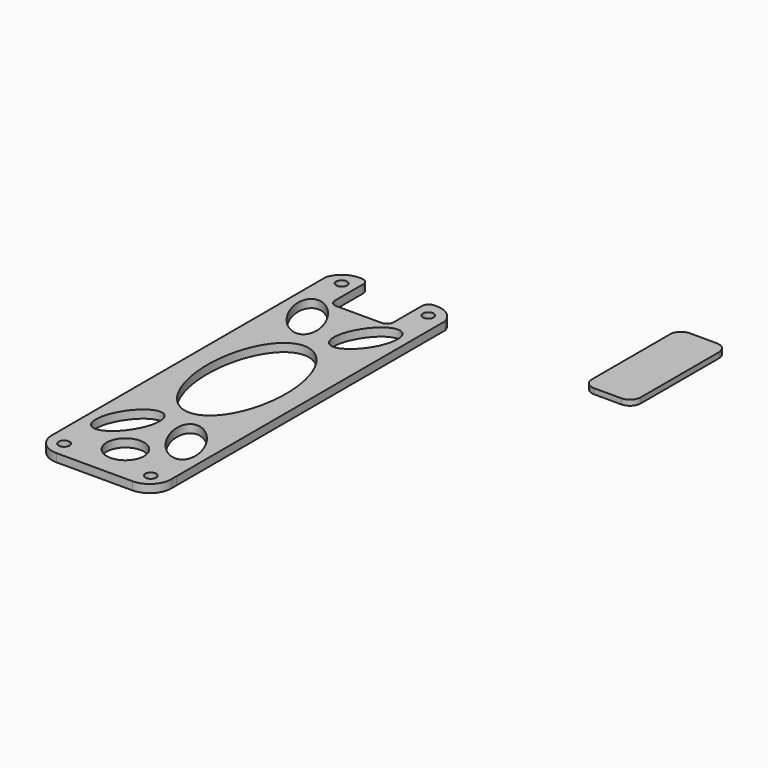
from build123d import *

# Parameters (mm, degrees)
F0_R     = 1
F0_R_2   = 3.4365293236
F1_DEPTH = 1.5
F3_DEPTH = 1


# Not quite as in the source:
# - ends of sketch curves that miss each other by under 0.0002 mm in the source are joined


with BuildPart() as f1:
    # F0 (on Top) → F1 (new body)
    with BuildSketch(Plane.XY):
        with BuildLine():
            Line((-6.6703559288, 34.8672945046), (-7.2344225406, 34.8672945046))
            ThreePointArc((-7.2344225406, 34.8672945046), (-9.5878669678, 34.0491231833), (-11.0004434851, 31.996628953))
            Line((-11.0004434851, 31.996628953), (-10.9999999994, -30.0032136791))
            Line((-10.9999999994, -30.0032136791), (-10.9999999994, -31.003371047))
            ThreePointArc((-10.9999999994, -31.003371047), (-9.8758814594, -33.9150302613), (-7.0020914712, -35.1327054954))
            Line((-7.0020914712, -35.1327054954), (6.8289959157, -35.1327054954))
            Line((6.8289959157, -35.1327054954), (7.0020914712, -35.1327054954))
            ThreePointArc((7.0020914712, -35.1327054954), (9.8758814594, -33.9150302613), (10.9999999994, -31.003371047))
            Line((10.9999999994, -31.003371047), (11, -30.0030563128))
            Line((11, -30.0030563128), (10.9995565132, 31.9969436856))
            Line((10.9995565132, 31.9969436856), (10.9995493379, 31.9996645259))
            ThreePointArc((10.9995493379, 31.9996645259), (9.5866084094, 34.0500821314), (7.2344225406, 34.8672945046))
            Line((7.2344225406, 34.8672945046), (6.6703559288, 34.8672945046))
            ThreePointArc((6.6703559288, 34.8672945046), (5.7859899934, 34.5009781401), (5.4196736289, 33.6166122047))
            Line((5.4196736289, 33.6166122047), (5.4196736289, 28.8547880611))
            Line((5.4196736289, 28.8547880611), (5.4196736289, 27.1179768046))
            ThreePointArc((5.4196736289, 27.1179768046), (5.0533572643, 26.2336108692), (4.1689913289, 25.8672945046))
            Line((4.1689913289, 25.8672945046), (-4.1689913289, 25.8672945046))
            ThreePointArc((-4.1689913289, 25.8672945046), (-5.0533572643, 26.2336108692), (-5.4196736289, 27.1179768046))
            Line((-5.4196736289, 27.1179768046), (-5.4196736289, 28.8547880611))
            Line((-5.4196736289, 28.8547880611), (-5.4196736289, 33.6166122047))
            ThreePointArc((-5.4196736289, 33.6166122047), (-5.7859899934, 34.5009781401), (-6.6703559288, 34.8672945046))
        make_face()
        with Locations((-7.9999999994, -32.1327054954)):
            Circle(F0_R, mode=Mode.SUBTRACT)
        with Locations((0, -27.9928222299)):
            Circle(F0_R_2, mode=Mode.SUBTRACT)
        with BuildLine():
            add(Edge.make_bspline(
                [(-2.5573940948, -15.9008428454), (-6.9030631327, -13.3373837718), (-8.9732737277, -21.8120776777), (-11.0434843227, -30.2867715836), (-4.6276046898, -24.3755367514), (1.7882749432, -18.4643019191), (-2.5573940948, -15.9008428454)],
                knots=[0, 0, 0, 2.0943951024, 2.0943951024, 4.1887902048, 4.1887902048, 6.2831853072, 6.2831853072, 6.2831853072], degree=2, weights=[1, 0.5, 1, 0.5, 1, 0.5, 1]))
        make_face(mode=Mode.SUBTRACT)
        with BuildLine():
            add(Edge.make_bspline(
                [(2.5573940948, -15.9008428454), (-1.7882749432, -18.4643019191), (4.6276046898, -24.3755367514), (11.0434843227, -30.2867715836), (8.9732737277, -21.8120776777), (6.9030631327, -13.3373837718), (2.5573940948, -15.9008428454)],
                knots=[0, 0, 0, 2.0943951024, 2.0943951024, 4.1887902048, 4.1887902048, 6.2831853072, 6.2831853072, 6.2831853072], degree=2, weights=[1, 0.5, 1, 0.5, 1, 0.5, 1]))
        make_face(mode=Mode.SUBTRACT)
        with Locations((8, -32.1327054954)):
            Circle(F0_R, mode=Mode.SUBTRACT)
        with BuildLine():
            add(Edge.make_bspline(
                [(0, -13.2964979857), (12.5666675431, -13.2964979857), (6.2833337715, 6.6482489929), (0, 26.5929959714), (-6.2833337715, 6.6482489929), (-12.5666675431, -13.2964979857), (0, -13.2964979857)],
                knots=[0, 0, 0, 2.0943951024, 2.0943951024, 4.1887902048, 4.1887902048, 6.2831853072, 6.2831853072, 6.2831853072], degree=2, weights=[1, 0.5, 1, 0.5, 1, 0.5, 1]))
        make_face(mode=Mode.SUBTRACT)
        with Locations((-8, 31.8672945046)):
            Circle(F0_R, mode=Mode.SUBTRACT)
        with BuildLine():
            add(Edge.make_bspline(
                [(-2.5573940948, 15.9008428454), (1.7882749432, 18.4643019191), (-4.6276046898, 24.3755367514), (-11.0434843227, 30.2867715836), (-8.9732737277, 21.8120776777), (-6.9030631327, 13.3373837718), (-2.5573940948, 15.9008428454)],
                knots=[0, 0, 0, 2.0943951024, 2.0943951024, 4.1887902048, 4.1887902048, 6.2831853072, 6.2831853072, 6.2831853072], degree=2, weights=[1, 0.5, 1, 0.5, 1, 0.5, 1]))
        make_face(mode=Mode.SUBTRACT)
        with BuildLine():
            add(Edge.make_bspline(
                [(2.5573940948, 15.9008428454), (6.9030631327, 13.3373837718), (8.9732737277, 21.8120776777), (11.0434843227, 30.2867715836), (4.6276046898, 24.3755367514), (-1.7882749432, 18.4643019191), (2.5573940948, 15.9008428454)],
                knots=[0, 0, 0, 2.0943951024, 2.0943951024, 4.1887902048, 4.1887902048, 6.2831853072, 6.2831853072, 6.2831853072], degree=2, weights=[1, 0.5, 1, 0.5, 1, 0.5, 1]))
        make_face(mode=Mode.SUBTRACT)
        with Locations((8, 31.8672945046)):
            Circle(F0_R, mode=Mode.SUBTRACT)
    extrude(amount=F1_DEPTH)


with BuildPart() as f3:
    # F2 (on Top) → F3 (new body)
    with BuildSketch(Plane.XY):
        with BuildLine():
            Line((45.2493974566, 51.8187274049), (40.2493974566, 51.8187274049))
            ThreePointArc((40.2493974566, 51.8187274049), (38.8351838943, 51.2329409672), (38.2493974566, 49.8187274049))
            Line((38.2493974566, 49.8187274049), (38.2493974566, 31.8187274049))
            ThreePointArc((38.2493974566, 31.8187274049), (38.8351838943, 30.4045138425), (40.2493974566, 29.8187274049))
            Line((40.2493974566, 29.8187274049), (45.2493974566, 29.8187274049))
            ThreePointArc((45.2493974566, 29.8187274049), (46.663611019, 30.4045138425), (47.2493974566, 31.8187274049))
            Line((47.2493974566, 31.8187274049), (47.2493974566, 49.8187274049))
            ThreePointArc((47.2493974566, 49.8187274049), (46.663611019, 51.2329409672), (45.2493974566, 51.8187274049))
        make_face()
    extrude(amount=F3_DEPTH)


solid = Compound([f1.part, f3.part])
